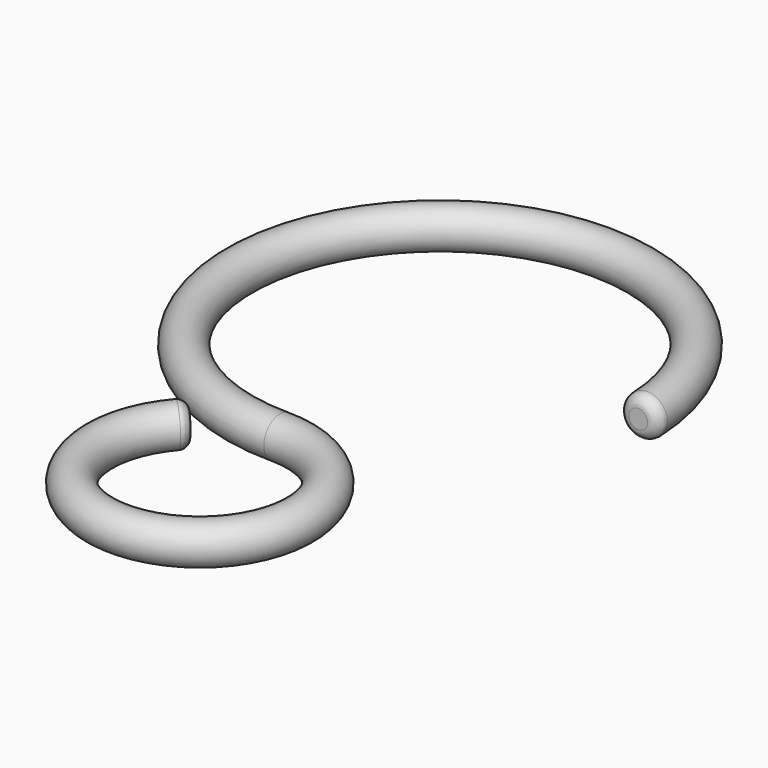
from build123d import *

# Parameters (mm, degrees)
F1_R = 1
F3_R = 0.4828427125
F4_R = 0.5311269837


with BuildPart() as f2:
    # F2: sweep along a path in F0
    with BuildLine(Plane.XY) as f2_path:
        ThreePointArc((9.9995049802, 9.9005005005), (-7.0358014826, 17.1061591241), (0, 0))
        ThreePointArc((0, 0), (1.8438696101, -9.6475956), (-3.4278241147, -1.3599420556))
    # F1 (on Right) → F2 (sweep)
    with BuildSketch(Plane.YZ):
        Circle(F1_R)
    sweep(path=f2_path.line)

    # F3
    f3_edges = [f2.edges().sort_by_distance(p)[0] for p in [
        (-2.742259, -2.087954, 0),
    ]]
    fillet(f3_edges, radius=F3_R)

    # F4
    f4_edges = [f2.edges().sort_by_distance(p)[0] for p in [
        (10.999455, 9.890551, 0),
    ]]
    fillet(f4_edges, radius=F4_R)


solid = f2.part
